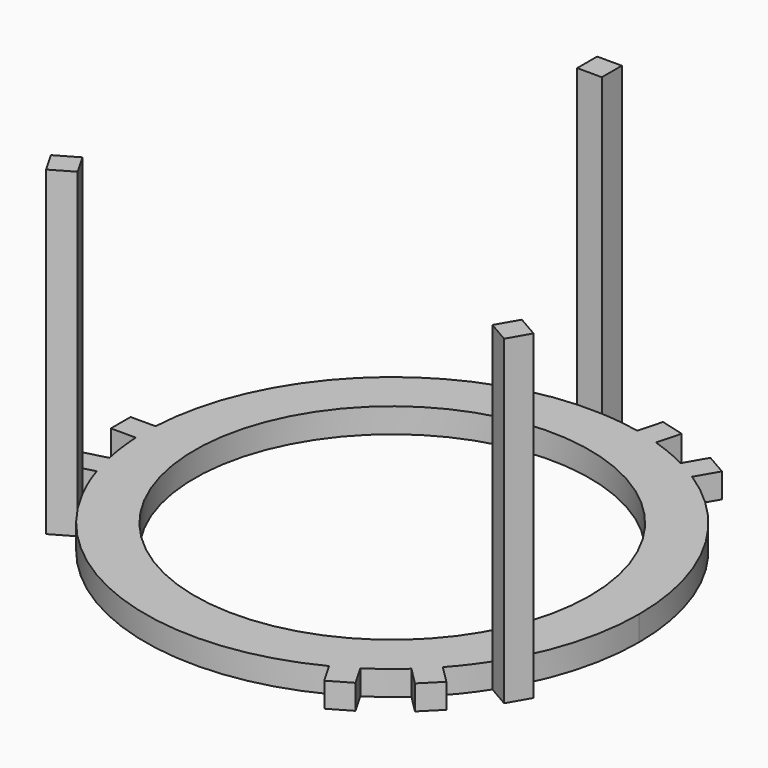
from build123d import *

# Parameters (mm, degrees)
F0_R     = 50.8
F1_DEPTH = 6.35
F2_W     = 6.35
F2_H     = 6.4294246715
F3_DEPTH = 76.2


# Not quite as in the source:
# - a feature names something its author has since deleted; it is built from what else it names


with BuildPart() as f1:
    # F0 (on Top) → F1 (new body)
    with BuildSketch(Plane.XY):
        with BuildLine():
            ThreePointArc((56.5113293571, -28.9606570072), (61.7281111576, -14.895982442), (63.5, 0))
            ThreePointArc((63.5, 0), (55.7694128237, 30.3648249344), (34.4599183213, 53.3363293571))
            Line((34.4599183213, 53.3363293571), (31.324630657, 47.9058518263))
            Line((31.324630657, 47.9058518263), (25.825369343, 51.0808518263))
            Line((25.825369343, 51.0808518263), (28.9606570072, 56.5113293571))
            ThreePointArc((28.9606570072, 56.5113293571), (24.3003979552, 58.6663503145), (19.4812672448, 60.4378211597))
            Line((19.4812672448, 60.4378211597), (17.8583229261, 54.3809105042))
            Line((17.8583229261, 54.3809105042), (11.7246939291, 56.0244114406))
            Line((11.7246939291, 56.0244114406), (13.3476382479, 62.0813220961))
            ThreePointArc((13.3476382479, 62.0813220961), (8.288413206, 62.9567486972), (3.175, 63.4205753285))
            Line((3.175, 63.4205753285), (3.175, 57.15))
            Line((3.175, 57.15), (-3.175, 57.15))
            Line((-3.175, 57.15), (-3.175, 63.4205753285))
            ThreePointArc((-3.175, 63.4205753285), (-44.9012806053, 44.9012806053), (-63.4205753285, 3.175))
            Line((-63.4205753285, 3.175), (-57.15, 3.175))
            Line((-57.15, 3.175), (-57.15, -3.175))
            Line((-57.15, -3.175), (-63.4205753285, -3.175))
            ThreePointArc((-63.4205753285, -3.175), (-62.9567486972, -8.288413206), (-62.0813220961, -13.3476382479))
            Line((-62.0813220961, -13.3476382479), (-56.0244114406, -11.7246939291))
            Line((-56.0244114406, -11.7246939291), (-54.3809105042, -17.8583229261))
            Line((-54.3809105042, -17.8583229261), (-60.4378211597, -19.4812672448))
            ThreePointArc((-60.4378211597, -19.4812672448), (-58.6663503145, -24.3003979552), (-56.5113293571, -28.9606570072))
            Line((-56.5113293571, -28.9606570072), (-51.0808518263, -25.825369343))
            Line((-51.0808518263, -25.825369343), (-47.9058518263, -31.324630657))
            Line((-47.9058518263, -31.324630657), (-53.3363293571, -34.4599183213))
            ThreePointArc((-53.3363293571, -34.4599183213), (-16.435009364, -61.3362899694), (28.9606570072, -56.5113293571))
            Line((28.9606570072, -56.5113293571), (25.825369343, -51.0808518263))
            Line((25.825369343, -51.0808518263), (31.324630657, -47.9058518263))
            Line((31.324630657, -47.9058518263), (34.4599183213, -53.3363293571))
            ThreePointArc((34.4599183213, -53.3363293571), (38.6563507421, -50.3779371085), (42.6000548513, -47.0901829118))
            Line((42.6000548513, -47.0901829118), (38.1660885145, -42.6562165751))
            Line((38.1660885145, -42.6562165751), (42.6562165751, -38.1660885145))
            Line((42.6562165751, -38.1660885145), (47.0901829118, -42.6000548513))
            ThreePointArc((47.0901829118, -42.6000548513), (50.3779371085, -38.6563507421), (53.3363293571, -34.4599183213))
            Line((53.3363293571, -34.4599183213), (47.9058518263, -31.324630657))
            Line((47.9058518263, -31.324630657), (51.0808518263, -25.825369343))
            Line((51.0808518263, -25.825369343), (56.5113293571, -28.9606570072))
        make_face()
        Circle(F0_R, mode=Mode.SUBTRACT)
        with BuildLine():
            ThreePointArc((-3.175, 63.4205753285), (0, 63.5), (3.175, 63.4205753285))
            Line((3.175, 63.4205753285), (3.175, 69.85))
            Line((3.175, 69.85), (-3.175, 69.85))
            Line((-3.175, 69.85), (-3.175, 63.4205753285))
        make_face()
        with BuildLine():
            Line((3.175, 57.15), (3.175, 63.4205753285))
            ThreePointArc((3.175, 63.4205753285), (0, 63.5), (-3.175, 63.4205753285))
            Line((-3.175, 63.4205753285), (-3.175, 57.15))
            Line((-3.175, 57.15), (3.175, 57.15))
        make_face()
        with BuildLine():
            Line((17.8583229261, 54.3809105042), (19.4812672448, 60.4378211597))
            ThreePointArc((19.4812672448, 60.4378211597), (16.435009364, 61.3362899694), (13.3476382479, 62.0813220961))
            Line((13.3476382479, 62.0813220961), (11.7246939291, 56.0244114406))
            Line((11.7246939291, 56.0244114406), (17.8583229261, 54.3809105042))
        make_face()
        with BuildLine():
            ThreePointArc((13.3476382479, 62.0813220961), (16.435009364, 61.3362899694), (19.4812672448, 60.4378211597))
            Line((19.4812672448, 60.4378211597), (21.1453247989, 66.6481684981))
            Line((21.1453247989, 66.6481684981), (15.0116958019, 68.2916694345))
            Line((15.0116958019, 68.2916694345), (13.3476382479, 62.0813220961))
        make_face()
        with BuildLine():
            ThreePointArc((28.9606570072, 56.5113293571), (31.75, 54.9926131403), (34.4599183213, 53.3363293571))
            Line((34.4599183213, 53.3363293571), (37.674630657, 58.9043744543))
            Line((37.674630657, 58.9043744543), (32.175369343, 62.0793744543))
            Line((32.175369343, 62.0793744543), (28.9606570072, 56.5113293571))
        make_face()
        with BuildLine():
            Line((31.324630657, 47.9058518263), (34.4599183213, 53.3363293571))
            ThreePointArc((34.4599183213, 53.3363293571), (31.75, 54.9926131403), (28.9606570072, 56.5113293571))
            Line((28.9606570072, 56.5113293571), (25.825369343, 51.0808518263))
            Line((25.825369343, 51.0808518263), (31.324630657, 47.9058518263))
        make_face()
        with BuildLine():
            Line((62.0793744543, -32.175369343), (56.5113293571, -28.9606570072))
            ThreePointArc((56.5113293571, -28.9606570072), (54.9926131403, -31.75), (53.3363293571, -34.4599183213))
            Line((53.3363293571, -34.4599183213), (58.9043744543, -37.674630657))
            Line((58.9043744543, -37.674630657), (62.0793744543, -32.175369343))
        make_face()
        with BuildLine():
            ThreePointArc((53.3363293571, -34.4599183213), (54.9926131403, -31.75), (56.5113293571, -28.9606570072))
            Line((56.5113293571, -28.9606570072), (51.0808518263, -25.825369343))
            Line((51.0808518263, -25.825369343), (47.9058518263, -31.324630657))
            Line((47.9058518263, -31.324630657), (53.3363293571, -34.4599183213))
        make_face()
        with BuildLine():
            Line((51.6364726961, -47.1463446356), (47.0901829118, -42.6000548513))
            ThreePointArc((47.0901829118, -42.6000548513), (44.9012806053, -44.9012806053), (42.6000548513, -47.0901829118))
            Line((42.6000548513, -47.0901829118), (47.1463446356, -51.6364726961))
            Line((47.1463446356, -51.6364726961), (51.6364726961, -47.1463446356))
        make_face()
        with BuildLine():
            ThreePointArc((42.6000548513, -47.0901829118), (44.9012806053, -44.9012806053), (47.0901829118, -42.6000548513))
            Line((47.0901829118, -42.6000548513), (42.6562165751, -38.1660885145))
            Line((42.6562165751, -38.1660885145), (38.1660885145, -42.6562165751))
            Line((38.1660885145, -42.6562165751), (42.6000548513, -47.0901829118))
        make_face()
        with BuildLine():
            ThreePointArc((28.9606570072, -56.5113293571), (31.75, -54.9926131403), (34.4599183213, -53.3363293571))
            Line((34.4599183213, -53.3363293571), (31.324630657, -47.9058518263))
            Line((31.324630657, -47.9058518263), (25.825369343, -51.0808518263))
            Line((25.825369343, -51.0808518263), (28.9606570072, -56.5113293571))
        make_face()
        with BuildLine():
            Line((37.674630657, -58.9043744543), (34.4599183213, -53.3363293571))
            ThreePointArc((34.4599183213, -53.3363293571), (31.75, -54.9926131403), (28.9606570072, -56.5113293571))
            Line((28.9606570072, -56.5113293571), (32.175369343, -62.0793744543))
            Line((32.175369343, -62.0793744543), (37.674630657, -58.9043744543))
        make_face()
        with BuildLine():
            Line((-58.9043744543, -37.674630657), (-53.3363293571, -34.4599183213))
            ThreePointArc((-53.3363293571, -34.4599183213), (-54.9926131403, -31.75), (-56.5113293571, -28.9606570072))
            Line((-56.5113293571, -28.9606570072), (-62.0793744543, -32.175369343))
            Line((-62.0793744543, -32.175369343), (-58.9043744543, -37.674630657))
        make_face()
        with BuildLine():
            ThreePointArc((-60.4378211597, -19.4812672448), (-61.3362899694, -16.435009364), (-62.0813220961, -13.3476382479))
            Line((-62.0813220961, -13.3476382479), (-68.2916694345, -15.0116958019))
            Line((-68.2916694345, -15.0116958019), (-66.6481684981, -21.1453247989))
            Line((-66.6481684981, -21.1453247989), (-60.4378211597, -19.4812672448))
        make_face()
        with BuildLine():
            ThreePointArc((-63.4205753285, -3.175), (-63.5, 0), (-63.4205753285, 3.175))
            Line((-63.4205753285, 3.175), (-69.85, 3.175))
            Line((-69.85, 3.175), (-69.85, -3.175))
            Line((-69.85, -3.175), (-63.4205753285, -3.175))
        make_face()
        with BuildLine():
            Line((-57.15, 3.175), (-63.4205753285, 3.175))
            ThreePointArc((-63.4205753285, 3.175), (-63.5, 0), (-63.4205753285, -3.175))
            Line((-63.4205753285, -3.175), (-57.15, -3.175))
            Line((-57.15, -3.175), (-57.15, 3.175))
        make_face()
        with BuildLine():
            Line((-56.0244114406, -11.7246939291), (-62.0813220961, -13.3476382479))
            ThreePointArc((-62.0813220961, -13.3476382479), (-61.3362899694, -16.435009364), (-60.4378211597, -19.4812672448))
            Line((-60.4378211597, -19.4812672448), (-54.3809105042, -17.8583229261))
            Line((-54.3809105042, -17.8583229261), (-56.0244114406, -11.7246939291))
        make_face()
        with BuildLine():
            ThreePointArc((-56.5113293571, -28.9606570072), (-54.9926131403, -31.75), (-53.3363293571, -34.4599183213))
            Line((-53.3363293571, -34.4599183213), (-47.9058518263, -31.324630657))
            Line((-47.9058518263, -31.324630657), (-51.0808518263, -25.825369343))
            Line((-51.0808518263, -25.825369343), (-56.5113293571, -28.9606570072))
        make_face()
    extrude(amount=F1_DEPTH)

    # F2 (on face) → F3 (join)
    with BuildSketch(Plane.XY.offset(6.35)):
        with Locations((0, 66.6352876643)):
            Rectangle(F2_W, F2_H)
        Polygon((62.0793744543, -32.175369343), (56.5113293571, -28.9606570072), (53.3363293571, -34.4599183213), (58.9043744543, -37.674630657), align=None)
        Polygon((-53.3363293571, -34.4599183213), (-56.5113293571, -28.9606570072), (-62.0793744543, -32.175369343), (-58.9043744543, -37.674630657), align=None)
    extrude(amount=F3_DEPTH)


solid = f1.part
